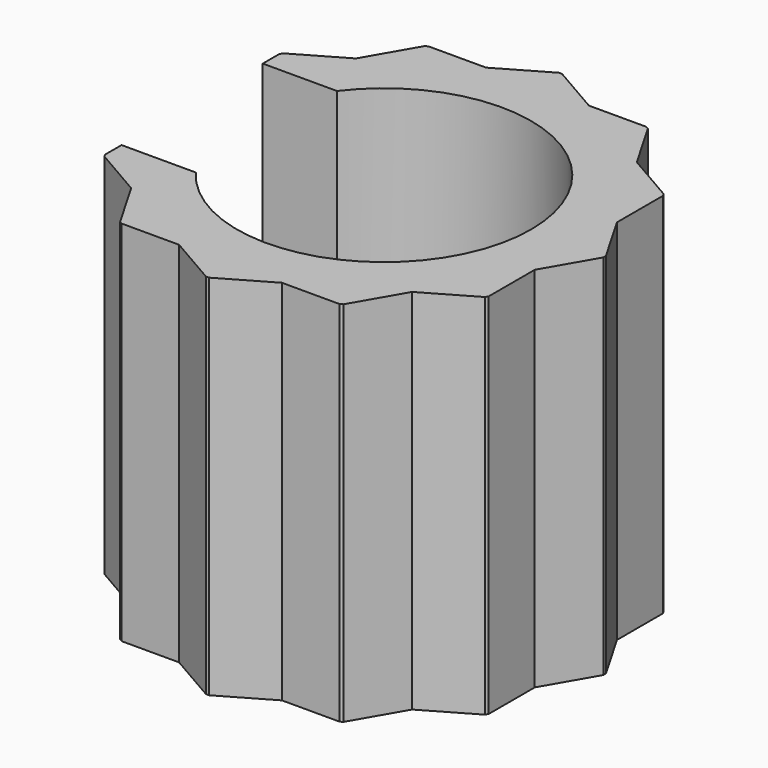
from build123d import *

# Parameters (mm, degrees)
F1_DEPTH = 12.5


# Not quite as in the source:
# - ends of sketch curves that miss each other by under 0.0002 mm in the source are joined


with BuildPart() as f1:
    # F0 (on Top) → F1 (new body, symmetric)
    with BuildSketch(Plane.XY):
        with BuildLine():
            ThreePointArc((14.9995966273, -0.1100046231), (14.9998991565, -0.0550026813), (15, 0))
            ThreePointArc((15, 0), (14.9998991565, 0.0550026813), (14.9995966273, 0.1100046231))
            Line((14.9995966273, 0.1100046231), (13.0450340373, 3.4954063355))
            Line((13.0450340373, 3.4954063355), (13.0450340373, 7.4045315155))
            ThreePointArc((13.0450340373, 7.4045315155), (12.9903810568, 7.5), (12.9350294143, 7.5950651118))
            Line((12.9350294143, 7.5950651118), (9.5496277018, 9.5496277018))
            Line((9.5496277018, 9.5496277018), (7.5950651118, 12.9350294143))
            ThreePointArc((7.5950651118, 12.9350294143), (7.5, 12.9903810568), (7.4045315155, 13.0450340373))
            Line((7.4045315155, 13.0450340373), (3.4954063355, 13.0450340373))
            Line((3.4954063355, 13.0450340373), (0.1100046231, 14.9995966273))
            ThreePointArc((0.1100046231, 14.9995966273), (0, 15), (-0.1100046231, 14.9995966273))
            Line((-0.1100046231, 14.9995966273), (-3.4954063355, 13.0450340373))
            Line((-3.4954063355, 13.0450340373), (-7.4045315155, 13.0450340373))
            ThreePointArc((-7.4045315155, 13.0450340373), (-7.5, 12.9903810568), (-7.5950651118, 12.9350294143))
            Line((-7.5950651118, 12.9350294143), (-9.5496277018, 9.5496277018))
            Line((-9.5496277018, 9.5496277018), (-12.9350294143, 7.5950651118))
            ThreePointArc((-12.9350294143, 7.5950651118), (-12.9903810568, 7.5), (-13.0450340373, 7.4045315155))
            Line((-13.0450340373, 7.4045315155), (-13.0450340373, 6))
            Line((-13.0450340373, 6), (-8, 6))
            ThreePointArc((-8, 6), (3.1622775895, 9.4868327685), (9.9999997765, 0))
            ThreePointArc((9.9999997765, 0), (3.1622775895, -9.4868327685), (-7.9999998212, -5.9999998659))
            Line((-7.9999998212, -5.9999998659), (-13.0450340373, -6))
            Line((-13.0450340373, -6), (-13.0450340373, -7.4045315155))
            ThreePointArc((-13.0450340373, -7.4045315155), (-12.9903810568, -7.5), (-12.9350294143, -7.5950651118))
            Line((-12.9350294143, -7.5950651118), (-9.5496277018, -9.5496277018))
            Line((-9.5496277018, -9.5496277018), (-7.5950651118, -12.9350294143))
            ThreePointArc((-7.5950651118, -12.9350294143), (-7.5, -12.9903810568), (-7.4045315155, -13.0450340373))
            Line((-7.4045315155, -13.0450340373), (-3.4954063355, -13.0450340373))
            Line((-3.4954063355, -13.0450340373), (-0.1100046231, -14.9995966273))
            ThreePointArc((-0.1100046231, -14.9995966273), (0, -15), (0.1100046231, -14.9995966273))
            Line((0.1100046231, -14.9995966273), (3.4954063355, -13.0450340373))
            Line((3.4954063355, -13.0450340373), (7.4045315155, -13.0450340373))
            ThreePointArc((7.4045315155, -13.0450340373), (7.5, -12.9903810568), (7.5950651118, -12.9350294143))
            Line((7.5950651118, -12.9350294143), (9.5496277018, -9.5496277018))
            Line((9.5496277018, -9.5496277018), (12.9350294143, -7.5950651118))
            ThreePointArc((12.9350294143, -7.5950651118), (12.9903810568, -7.5), (13.0450340373, -7.4045315155))
            Line((13.0450340373, -7.4045315155), (13.0450340373, -3.4954063355))
            Line((13.0450340373, -3.4954063355), (14.9995966273, -0.1100046231))
        make_face()
    extrude(amount=F1_DEPTH, both=True)


solid = f1.part
